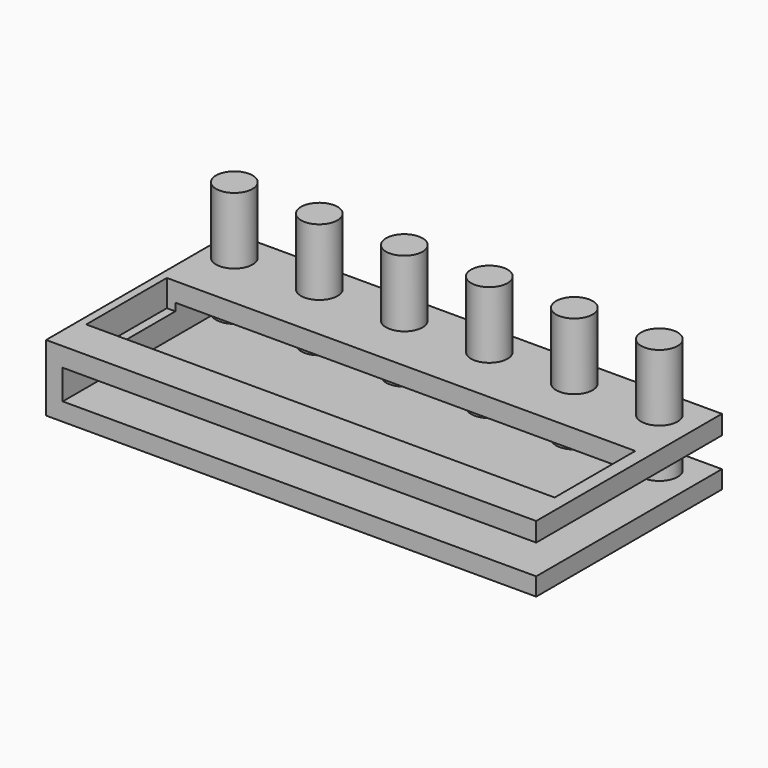
from build123d import *

# Parameters (mm, degrees)
F0_R     = 1.3710803726
F1_DEPTH = 10
F0_W     = 36.7866121233
F0_H     = 17.4243357033
F2_DEPTH = 5
F3_W     = 35.1581810974
F3_H     = 7.5634159148
F4_DEPTH = 2
F6_DEPTH = 25


with BuildPart() as f1:
    # F0 (on Top) → F1 (new body)
    with BuildSketch(Plane.XY):
        with Locations((8.4812443238, 15.0325801224)):
            Circle(F0_R)
    extrude(amount=F1_DEPTH)


with BuildPart() as f1b:
    # F0 (on Top) → F1, piece 2 (new body)
    with BuildSketch(Plane.XY):
        with Locations((14.8622810375, 15.0325801224)):
            Circle(F0_R)
    extrude(amount=F1_DEPTH)


with BuildPart() as f1c:
    # F0 (on Top) → F1, piece 3 (new body)
    with BuildSketch(Plane.XY):
        with Locations((21.2433177512, 15.0325801224)):
            Circle(F0_R)
    extrude(amount=F1_DEPTH)


with BuildPart() as f1d:
    # F0 (on Top) → F1, piece 4 (new body)
    with BuildSketch(Plane.XY):
        with Locations((27.6243544649, 15.0325801224)):
            Circle(F0_R)
    extrude(amount=F1_DEPTH)


with BuildPart() as f1e:
    # F0 (on Top) → F1, piece 5 (new body)
    with BuildSketch(Plane.XY):
        with Locations((34.0053911787, 15.0325801224)):
            Circle(F0_R)
    extrude(amount=F1_DEPTH)


with BuildPart() as f1f:
    # F0 (on Top) → F1, piece 6 (new body)
    with BuildSketch(Plane.XY):
        with Locations((2.1002076101, 15.0325801224)):
            Circle(F0_R)
    extrude(amount=F1_DEPTH)


with BuildPart() as f2:
    # F0 (on Top) → F2 (new body)
    with BuildSketch(Plane.XY):
        with Locations((18.3933060616, 8.7121678516)):
            Rectangle(F0_W, F0_H)
        with Locations((2.1002076101, 15.0325801224)):
            Circle(F0_R, mode=Mode.SUBTRACT)
        with Locations((8.4812443238, 15.0325801224)):
            Circle(F0_R, mode=Mode.SUBTRACT)
        with Locations((14.8622810375, 15.0325801224)):
            Circle(F0_R, mode=Mode.SUBTRACT)
        with Locations((21.2433177512, 15.0325801224)):
            Circle(F0_R, mode=Mode.SUBTRACT)
        with Locations((27.6243544649, 15.0325801224)):
            Circle(F0_R, mode=Mode.SUBTRACT)
        with Locations((34.0053911787, 15.0325801224)):
            Circle(F0_R, mode=Mode.SUBTRACT)
    extrude(amount=F2_DEPTH)

    # F3 (on face) → F4 (cut)
    with BuildSketch(Plane.XY.offset(5)):
        with Locations((18.1877680589, 6.7874193192)):
            Rectangle(F3_W, F3_H)
    extrude(amount=-F4_DEPTH, mode=Mode.SUBTRACT)

    # F5 (on face) → F6 (cut)
    with BuildSketch(Plane.XZ):
        Polygon((1.2501757592, 3.5718409345), (1.2501757592, 1.3440612238), (36.7866121233, 1.3440612238), (37.6002937555, 1.3440612238), (37.6002937555, 3.5718409345), align=None)
    extrude(amount=-F6_DEPTH, mode=Mode.SUBTRACT)


solid = Compound([f1.part, f1b.part, f1c.part, f1d.part, f1e.part, f1f.part, f2.part])
